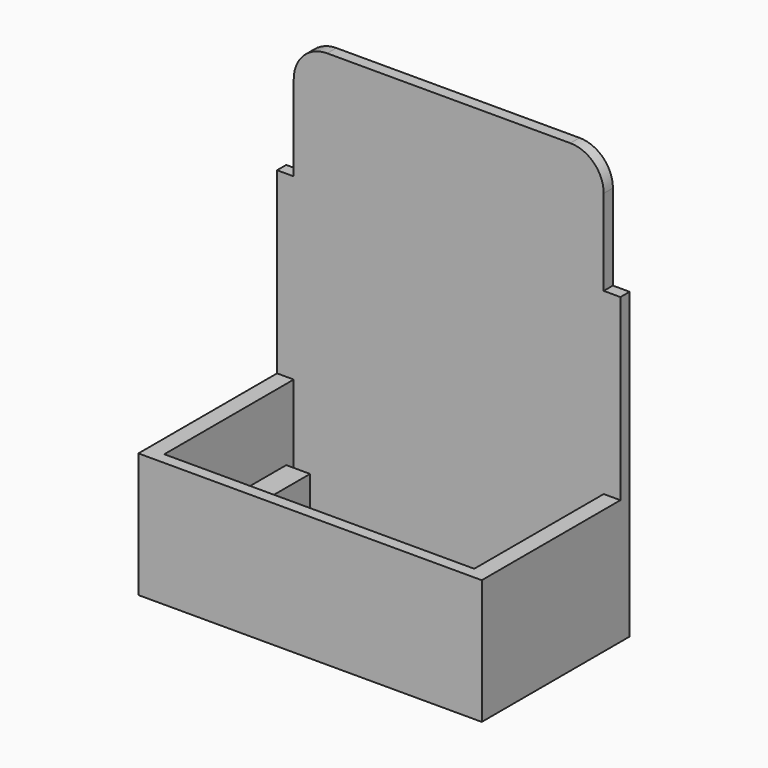
from build123d import *

# Parameters (mm, degrees)
F0_W          = 182.88
F0_H          = 98.425
F1_DEPTH      = 2.9464
F2_W          = 165.1
F2_H          = 6.1169746459
F3_DEPTH      = 63.5
F4_W          = 182.88
F4_H          = 6.1169746459
F5_DEPTH      = 95.25
F6_W          = 165.1
F6_H          = 6.1169746459
F7_DEPTH      = 63.5
F8_R          = 17.78
F9_W          = 101.6
F9_H          = 50.8
F10_DEPTH     = 0.254
F11_W         = 12.7
F11_H         = 76.2
F12_DEPTH     = 25.4
F13_W         = 76.2
F13_H         = 22.225
F14_DEPTH     = 12.7
F15_TEXT_SIZE = 20.8064603309
F16_DEPTH     = 0.254


# Not quite as in the source:
# - Text() gives the source's letters only with a copy of the font that has no kerning and outlines rounded to 1/6400 em; it was checked with that copy


with BuildPart() as f1:
    # F0 (on Top) → F1 (new body)
    with BuildSketch(Plane.XY):
        Rectangle(F0_W, F0_H)
    extrude(amount=F1_DEPTH)

    # F2 (on face) → F3 (join)
    with BuildSketch(Plane.XY.offset(2.9464)):
        Polygon((-82.55, 49.2125), (-91.44, 49.2125), (-91.44, -49.2125), (-82.55, -49.2125), (-82.55, -43.0955253541), (-82.55, 43.0955253541), align=None)
        with Locations((0, 46.1540126771)):
            Rectangle(F2_W, F2_H)
        Polygon((91.44, 49.2125), (82.55, 49.2125), (82.55, 43.0955253541), (82.55, -43.0955253541), (82.55, -49.2125), (91.44, -49.2125), align=None)
        with Locations((0, -46.1540126771)):
            Rectangle(F2_W, F2_H)
    extrude(amount=F3_DEPTH)

    # F4 (on face) → F5 (join)
    with BuildSketch(Plane.XY.offset(66.4464)):
        with Locations((0, 46.1540126771)):
            Rectangle(F4_W, F4_H)
    extrude(amount=F5_DEPTH)

    # F6 (on face) → F7 (join)
    with BuildSketch(Plane.XY.offset(161.6964)):
        with Locations((0, 46.1540126771)):
            Rectangle(F6_W, F6_H)
    extrude(amount=F7_DEPTH)

    # F8
    f8_edges = [f1.edges().sort_by_distance(p)[0] for p in [
        (-82.55, 46.154013, 225.1964),
        (82.55, 46.154013, 225.1964),
    ]]
    fillet(f8_edges, radius=F8_R)

    # F9 (on face) → F10 (join)
    with BuildSketch(Plane(origin=(0, 49.2125, 0), x_dir=(-1, 0, 0), z_dir=(0, 1, 0))):
        with Locations((0, 114.0714)):
            Rectangle(F9_W, F9_H)
    extrude(amount=F10_DEPTH)

    # F11 (on face) → F12 (join)
    with BuildSketch(Plane.XY.offset(2.9464)):
        with Locations((-76.2, 0)):
            Rectangle(F11_W, F11_H)
    extrude(amount=F12_DEPTH)

    # F13 (on face) → F14 (join)
    with BuildSketch(Plane.XY.offset(2.9464)):
        with Locations((44.45, -28.493218106)):
            Rectangle(F13_W, F13_H)
    extrude(amount=F14_DEPTH)

    # F15 (on face) → F16 (join)
    with BuildSketch(Plane(origin=(0, 49.4665, 0), x_dir=(-1, 0, 0), z_dir=(0, 1, 0))):
        with Locations(Location((30.7481141451, 123.0268701911), (0, 0, -180))):
            Text('LABEL', F15_TEXT_SIZE, font='Open Sans', text_align=(TextAlign.LEFT, TextAlign.BOTTOM))
    extrude(amount=F16_DEPTH)


solid = f1.part
